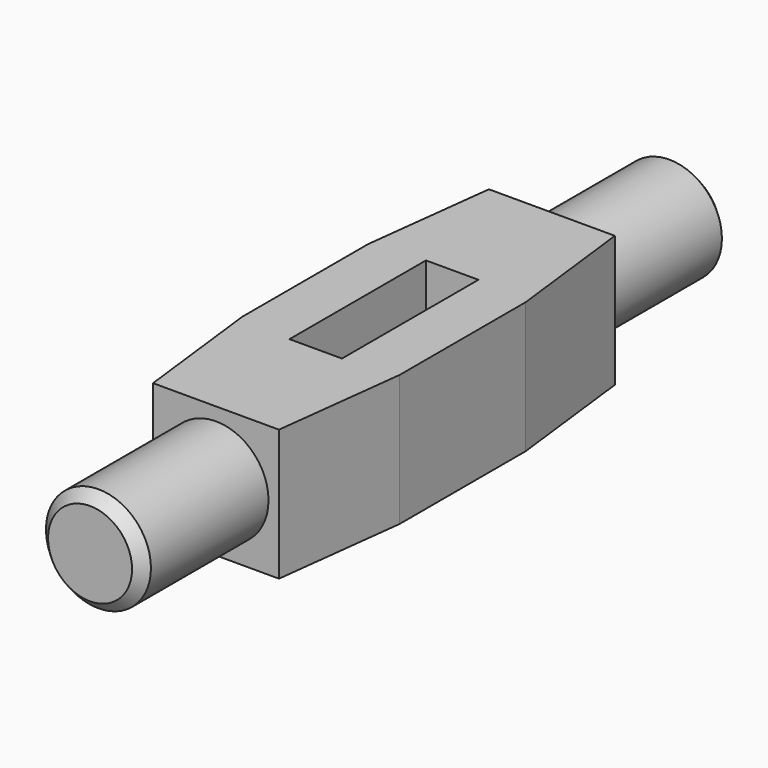
from build123d import *

# Parameters (mm, degrees)
F1_DEPTH = 12.5
F2_R     = 10
F3_DEPTH = 30
F4_SIZE  = 2
F5_W     = 10
F5_H     = 32.5
F6_DEPTH = 25


# Not quite as in the source:
# - a pattern or mirror of a feature is missing from the dataset's text; its kind, count and spacing are read off the source's solid


with BuildPart() as f1:
    # F0 (on Top) → F1 (new body, symmetric)
    with BuildSketch(Plane.XY):
        Polygon((-15, -15), (-12, -40), (12, -40), (15, -15), (15, 15), (12, 40), (-12, 40), (-15, 15), align=None)
    extrude(amount=F1_DEPTH, both=True)

    # F2 (on face) → F3 (join)
    with BuildSketch(Plane.XZ.offset(40)):
        Circle(F2_R)
    f3 = extrude(amount=F3_DEPTH)

    # F3_copies: F3 across plane
    add(f3.mirror(Plane.ZX))

    # F4
    f4_edges = [f1.edges().sort_by_distance(p)[0] for p in [
        (-10, -70, 0),
        (-10, 70, 0),
    ]]
    chamfer(f4_edges, length=F4_SIZE)

    # F5 (on face) → F6 (cut)
    with BuildSketch(Plane.XY.offset(12.5)):
        Rectangle(F5_W, F5_H)
    extrude(amount=-F6_DEPTH, mode=Mode.SUBTRACT)


solid = f1.part
